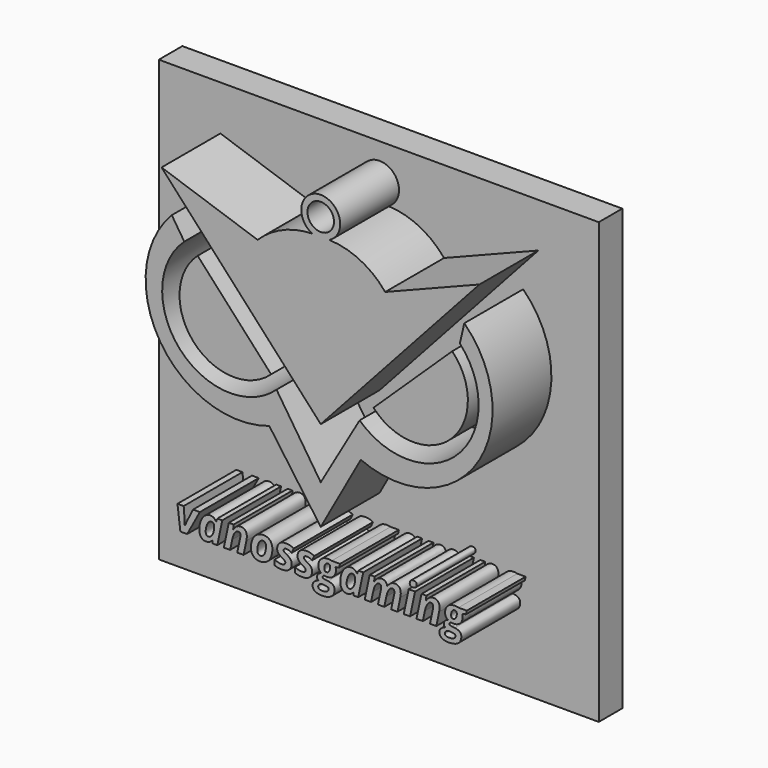
from build123d import *

# Parameters (mm, degrees)
F1_DEPTH      = 25
F3_DEPTH      = 25
F4_R          = 6.613392665
F5_DEPTH      = 25
F6_R          = 4.517131025
F7_DEPTH      = 25.3
F8_W          = 149.5320498943
F8_H          = 149.5320498943
F9_DEPTH      = 10
F11_DEPTH     = 25
F13_TEXT_SIZE = 14.6483257421
F14_DEPTH     = 25


# Not quite as in the source:
# - Text() gives the source's letters only with a copy of the font that has no kerning and outlines rounded to 1/6400 em; it was checked with that copy


with BuildPart() as f1:
    # F0 (on Front) → F1 (new body)
    with BuildSketch(Plane.XZ):
        with BuildLine():
            Line((-21.4529354125, 48.1679104269), (-54.1053828468, 59.2325731587))
            Line((-54.1053828468, 59.2325731587), (0, 0))
            Line((0, 0), (53.9712003756, 59.3548625305))
            Line((53.9712003756, 59.3548625305), (21.9099405086, 46.6792879186))
            ThreePointArc((21.9099405086, 46.6792879186), (12.1039610804, 54.0391816056), (0, 55.9935085475))
            ThreePointArc((0, 55.9935085475), (-11.5810583776, 54.4234669601), (-21.4529354125, 48.1679104269))
        make_face()
    extrude(amount=F1_DEPTH)

    # F4 (on Front) → F5 (join)
    with BuildSketch(Plane.XZ):
        with Locations((0, 62.017288059)):
            Circle(F4_R)
    extrude(amount=F5_DEPTH)

    # F6 (on Front) → F7 (cut)
    with BuildSketch(Plane.XZ):
        with Locations((0, 62.017288059)):
            Circle(F6_R)
    extrude(amount=F7_DEPTH, mode=Mode.SUBTRACT)


with BuildPart() as f3:
    # F2 (on Front) → F3 (new body)
    with BuildSketch(Plane.XZ):
        with BuildLine():
            Line((-16.8619342148, 9.4287525862), (-41.8317876756, 36.7854163051))
            ThreePointArc((-41.8317876756, 36.7854163051), (-43.1633315618, 10.4960712685), (-16.8619342148, 9.4287525862))
        make_face()
    extrude(amount=F3_DEPTH)


with BuildPart() as f3b:
    # F2 (on Front) → F3, piece 2 (new body)
    with BuildSketch(Plane.XZ):
        with BuildLine():
            ThreePointArc((17.9279092699, 10.7540665194), (44.2904121185, 9.9868598207), (44.6926992541, 36.3574557112))
            Line((44.6926992541, 36.3574557112), (17.9279092699, 10.7540665194))
        make_face()
    extrude(amount=F3_DEPTH)


with BuildPart() as f9:
    # F8 (on Front) → F9 (new body)
    with BuildSketch(Plane.XZ):
        with Locations((-0.2656020224, -0.2655982971)):
            Rectangle(F8_W, F8_H)
    extrude(amount=-F9_DEPTH)

    # F10 (on face) → F11 (join)
    with BuildSketch(Plane.XZ):
        with BuildLine():
            ThreePointArc((-15.0253018364, 5.4301102646), (-47.7898613192, 6.7744474075), (-46.3709358165, 39.5358614624))
            Line((-46.3709358165, 39.5358614624), (-50.6230257452, 46.0752695799))
            ThreePointArc((-50.6230257452, 46.0752695799), (-54.5703943434, 6.9278189627), (-17.4867038678, -6.2214969657))
            Line((-17.4867038678, -6.2214969657), (0, -30.7291521488))
            Line((0, -30.7291521488), (13.6082712561, -6.2214969657))
            ThreePointArc((13.6082712561, -6.2214969657), (52.949723932, 5.293938228), (48.7978376719, 46.0752695799))
            Line((48.7978376719, 46.0752695799), (47.2873022702, 39.5358614624))
            ThreePointArc((47.2873022702, 39.5358614624), (46.6061064984, 6.1311051567), (13.20175981, 5.4301102646))
            Line((13.20175981, 5.4301102646), (0, -17.3898860812))
            Line((0, -17.3898860812), (-15.0253018364, 5.4301102646))
        make_face()
    extrude(amount=F11_DEPTH)


with BuildPart() as f1_1:
    add(f1.part)

    # F12: union F3, F3b, F9
    add(f3.part)
    add(f3b.part)
    add(f9.part)

    # F13 (on face) → F14 (join)
    with BuildSketch(Plane.XZ):
        with Locations((-49.4238849594, -47.6528499881)):
            Text('vanossgaming', F13_TEXT_SIZE, font='Open Sans', font_style=FontStyle.BOLDITALIC, text_align=(TextAlign.LEFT, TextAlign.BOTTOM))
    extrude(amount=F14_DEPTH)


solid = f1_1.part
